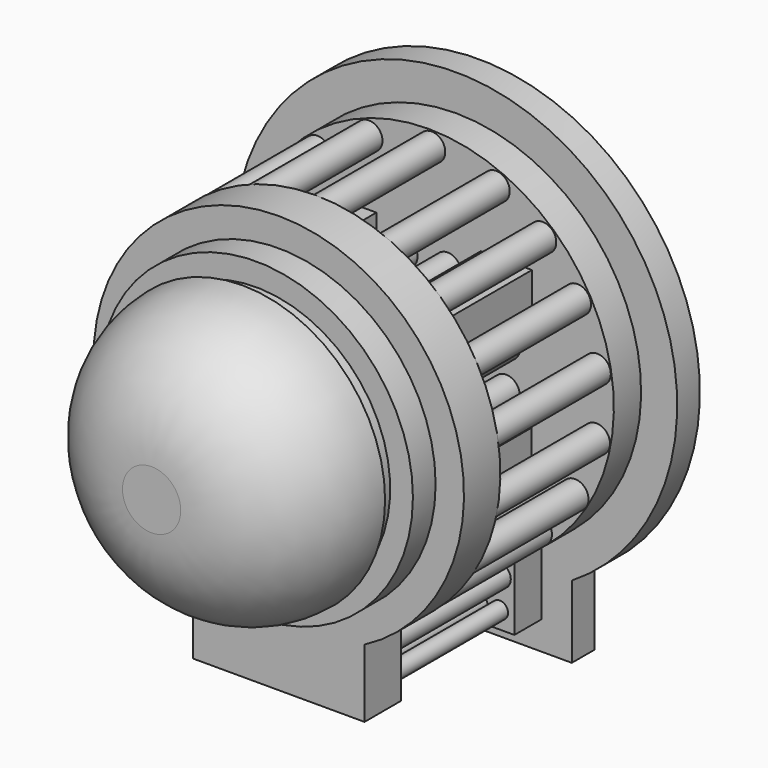
from build123d import *

# Parameters (mm, degrees)
F1_DEPTH  = 25.4
F2_R      = 25.39999
F3_R      = 30.0176409496
F4_DEPTH  = 3.81
F5_R      = 35.0976409496
F6_DEPTH  = 6.35
F7_R      = 35.0976409496
F8_DEPTH  = 10.16
F9_DEPTH  = 10.16
F10_W     = 38.3836512671
F10_H     = 10.16
F11_DEPTH = 15.24
F12_R     = 3.0425051658
F13_DEPTH = 31.75
F12_R_2   = 1.8599906357
F12_R_3   = 2.469076523
F12_R_4   = 2.4371339636
F12_W     = 11.43
F12_H     = 11.43
F15_DEPTH = 7.62
F18_DEPTH = 6.35


# Not quite as in the source:
# - a fillet or chamfer is up to 0.001 mm smaller than in the source, because OpenCascade refuses the exact size


with BuildPart() as f1:
    # F0 (on Front) → F1 (new body)
    with BuildSketch(Plane.XZ):
        with BuildLine():
            ThreePointArc((-51.3157695532, 20.9789809584), (-28.7430536644, 30.3289060191), (-19.3931286036, 52.9016219079))
            ThreePointArc((-19.3931286036, 52.9016219079), (-73.888485442, 75.4743377968), (-51.3157695532, 20.9789809584))
        make_face()
    extrude(amount=F1_DEPTH)

    # F2 (radius 25.4 in the source; OpenCascade refuses exactly that, so slightly less here)
    f2_edges = [f1.edges().sort_by_distance(p)[0] for p in [
        (-51.31577, -25.4, 84.824263),
    ]]
    fillet(f2_edges, radius=F2_R)

    # F3 (on face) → F4 (join)
    with BuildSketch(Plane(origin=(0, 0, 0), x_dir=(-1, 0, 0), z_dir=(0, 1, 0))):
        with Locations((51.3157695532, 52.9016219079)):
            Circle(F3_R)
    extrude(amount=F4_DEPTH)

    # F5 (on face) → F6 (join)
    with BuildSketch(Plane(origin=(0, 3.81, 0), x_dir=(-1, 0, 0), z_dir=(0, 1, 0))):
        with Locations((51.3157695532, 52.9016219079)):
            Circle(F5_R)
    extrude(amount=F6_DEPTH)



with BuildPart() as f8:
    # F7 (on face) → F8 (new body)
    with BuildSketch(Plane(origin=(0, 10.16, 0), x_dir=(-1, 0, 0), z_dir=(0, 1, 0))):
        with BuildLine():
            Line((32.1239439196, 16.1649812187), (70.5075951867, 16.1649812187))
            ThreePointArc((70.5075951867, 16.1649812187), (51.3157695532, 94.3492628575), (32.1239439196, 16.1649812187))
        make_face()
        with Locations((51.3157695532, 52.9016219079)):
            Circle(F7_R, mode=Mode.SUBTRACT)
    extrude(amount=F8_DEPTH)


with BuildPart() as f1_1:
    add(f1.part)

    add(f8.part)  # F9 merges F8
    # F7 (on face) → F9 (join)
    with BuildSketch(Plane(origin=(0, 10.16, 0), x_dir=(-1, 0, 0), z_dir=(0, 1, 0))):
        with Locations((51.3157695532, 52.9016219079)):
            Circle(F7_R)
    extrude(amount=F9_DEPTH)

    # F10 (on face) → F11 (join)
    with BuildSketch(Plane(origin=(0, 0, 16.1649812187), x_dir=(1, 0, 0), z_dir=(0, 0, -1))):
        with Locations((-51.3157695532, -15.24)):
            Rectangle(F10_W, F10_H)
    extrude(amount=F11_DEPTH)

    # F12 (on face) → F13, piece 2 (join)
    with BuildSketch(Plane(origin=(0, 20.32, 0), x_dir=(-1, 0, 0), z_dir=(0, 1, 0))):
        with Locations((67.4533173442, 4.8855347559)):
            Circle(F12_R_2)
        with Locations((35.3975147009, 4.8855352215)):
            Circle(F12_R_2)
        with Locations((39.9559102952, 4.8855347559)):
            Circle(F12_R_2)
        with Locations((44.3672593683, 4.8855361529)):
            Circle(F12_R_2)
        with Locations((49.0726977587, 4.8855366185)):
            Circle(F12_R_2)
        with Locations((53.6310952157, 4.8855361529)):
            Circle(F12_R_2)
        with Locations((58.0424424261, 4.8855347559)):
            Circle(F12_R_2)
        with Locations((62.6008361578, 4.8855366185)):
            Circle(F12_R_2)
        with Locations((35.3975147009, 11.7231269833)):
            Circle(F12_R_3)
        with Locations((67.4533173442, 11.7966495454)):
            Circle(F12_R_4)
        with Locations((13.5955894366, 59.4231709838)):
            Circle(F12_R)
        with Locations((50.6292656064, 91.1249816418)):
            Circle(F12_R)
        with Locations((18.5757915024, 33.1017822027)):
            Circle(F12_R)
        with Locations((25.7929724175, 81.4013928175)):
            Circle(F12_R)
        with Locations((89.0821111389, 59.1946728528)):
            Circle(F12_R)
        with Locations((84.0856006835, 33.2405753434)):
            Circle(F12_R)
        with Locations((76.2026160955, 81.9760784507)):
            Circle(F12_R)
        with Locations((36.2023725174, 88.0633927882)):
            Circle(F12_R)
        with Locations((88.8045257889, 45.3154779971)):
            Circle(F12_R)
        with Locations((18.0206210352, 71.6859512031)):
            Circle(F12_R)
        with Locations((13.761004433, 45.646622777)):
            Circle(F12_R)
        with Locations((64.6823644638, 88.7463241816)):
            Circle(F12_R)
        with Locations((84.7154408693, 71.5908780694)):
            Circle(F12_R)
        with Locations((26.7645169515, 23.525133729)):
            Circle(F12_R)
        with Locations((76.0732889175, 23.7615462393)):
            Circle(F12_R)
        with Locations((68.7132014135, 68.4635355137)):
            Rectangle(F12_W, F12_H)
        with Locations((33.9833064711, 37.3775935507)):
            Rectangle(F12_W, F12_H)
        with Locations((33.9119490236, 68.4635355137)):
            Rectangle(F12_W, F12_H)
        with Locations((68.7132014135, 37.3397083022)):
            Rectangle(F12_W, F12_H)
        with Locations((33.9833064711, 48.6564002931)):
            Circle(F12_R)
        with Locations((33.9119490236, 57.7810369432)):
            Circle(F12_R)
        with Locations((56.8348169327, 68.4635355137)):
            Circle(F12_R)
        with Locations((68.7132014135, 57.3359318078)):
            Circle(F12_R)
        with Locations((68.7132014135, 48.6564002931)):
            Circle(F12_R)
        with Locations((55.7220578194, 37.3397083022)):
            Circle(F12_R)
        with Locations((47.0425225794, 68.4635355137)):
            Circle(F12_R)
        with Locations((45.2621094882, 37.3775935507)):
            Circle(F12_R)
    extrude(amount=F13_DEPTH)

    # F14 (on face) → F15 (join)
    with BuildSketch(Plane(origin=(0, 52.07, 0), x_dir=(-1, 0, 0), z_dir=(0, 1, 0))):
        with BuildLine():
            Line((70.5171748996, 16.2905004551), (70.5051029675, 16.2905004551))
            ThreePointArc((70.5051029675, 16.2905004551), (51.313277334, 94.474782094), (32.1214517004, 16.2905004551))
            Line((32.1214517004, 16.2905004551), (32.1214517004, 1.0184145067))
            Line((32.1214517004, 1.0184145067), (70.5171748996, 1.0184145067))
            Line((70.5171748996, 1.0184145067), (70.5171748996, 16.2905004551))
        make_face()
    extrude(amount=F15_DEPTH)

    # F17 (on face) → F18 (join)
    with BuildSketch(Plane(origin=(0, 59.69, 0), x_dir=(-1, 0, 0), z_dir=(0, 1, 0))):
        with BuildLine():
            Line((77.230297029, -5.3806910291), (77.230297029, 10.8189785437))
            ThreePointArc((77.230297029, 10.8189785437), (51.3255716567, 102.5571396186), (25.3753070366, 10.8318499752))
            Line((25.3753070366, 10.8318499752), (25.3753070366, -5.3806910291))
            Line((25.3753070366, -5.3806910291), (77.230297029, -5.3806910291))
        make_face()
    extrude(amount=F18_DEPTH)


with BuildPart() as f13:
    # F12 (on face) → F13 (new body)
    with BuildSketch(Plane(origin=(0, 20.32, 0), x_dir=(-1, 0, 0), z_dir=(0, 1, 0))):
        with Locations((853.825874161, 233.101002872)):
            Circle(F12_R)
    extrude(amount=F13_DEPTH)


solid = f1_1.part
